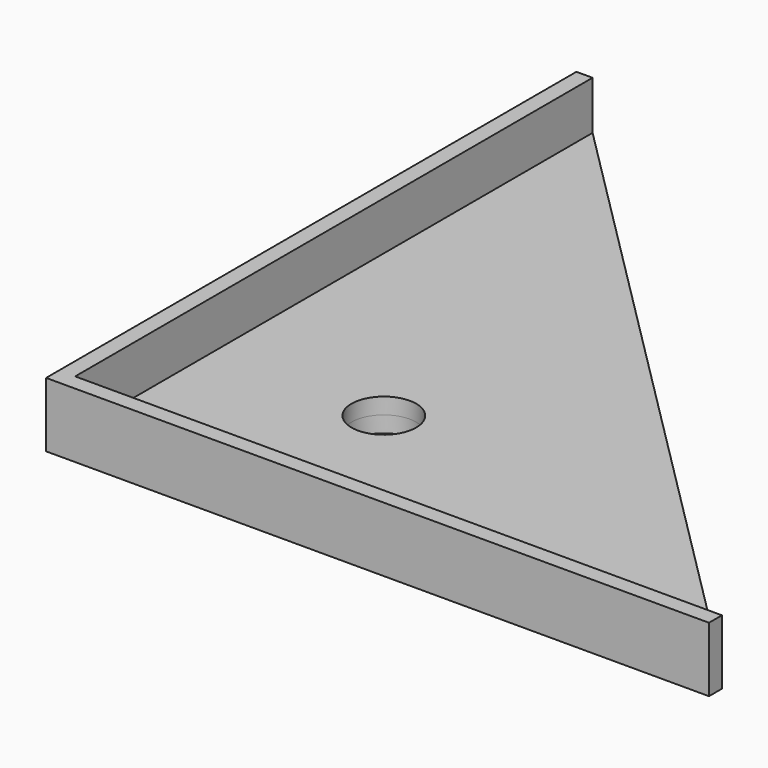
from build123d import *

# Parameters (mm, degrees)
F0_R     = 9.525
F0_R_2   = 6.35
F1_DEPTH = 3.175
F2_DEPTH = 12.7
F3_DEPTH = 3.175


# Not quite as in the source:
# - a feature names something its author has since deleted; it is built from what else it names


with BuildPart() as f1:
    # F0 (on Top) → F1 (new body)
    with BuildSketch(Plane.XY):
        Polygon((0, 127), (0, 0), (127, 0), align=None)
        with Locations((33.6748659611, 33.6748659611)):
            Circle(F0_R, mode=Mode.SUBTRACT)
        Polygon((127, 0), (0, 0), (0, 127), (-3.175, 127), (-3.175, -3.175), (127, -3.175), align=None)
        with Locations((33.6748659611, 33.6748659611)):
            Circle(F0_R)
        with Locations((33.6748659611, 33.6748659611)):
            Circle(F0_R_2, mode=Mode.SUBTRACT)
    extrude(amount=F1_DEPTH)

    # F0 (on Top) → F2 (join)
    with BuildSketch(Plane.XY):
        Polygon((127, 0), (0, 0), (0, 127), (-3.175, 127), (-3.175, -3.175), (127, -3.175), align=None)
    extrude(amount=F2_DEPTH)

    # F0 (on Top) → F3 (join)
    with BuildSketch(Plane.XY):
        with Locations((33.6748659611, 33.6748659611)):
            Circle(F0_R)
        with Locations((33.6748659611, 33.6748659611)):
            Circle(F0_R_2, mode=Mode.SUBTRACT)
    extrude(amount=-F3_DEPTH)


solid = f1.part
